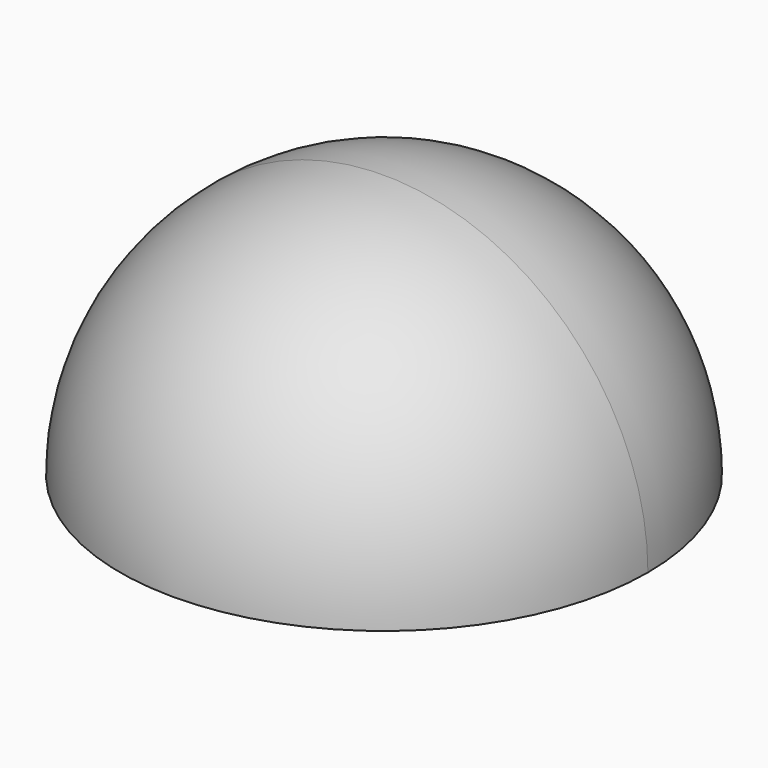
from build123d import *

# Parameters (mm, degrees)
F1_ANGLE = 180


with BuildPart() as f1:
    # F0 (on Top) → F1 (revolve)
    with BuildSketch(Plane.XY):
        with BuildLine():
            ThreePointArc((0, -31.75), (22.4506403027, -22.4506403027), (31.75, 0))
            ThreePointArc((31.75, 0), (22.4506403027, 22.4506403027), (0, 31.75))
            Line((0, 31.75), (0, 25.4))
            ThreePointArc((0, 25.4), (17.9605122421, 17.9605122421), (25.4, 0))
            ThreePointArc((25.4, 0), (17.9605122421, -17.9605122421), (0, -25.4))
            Line((0, -25.4), (0, -31.75))
        make_face()
    revolve(axis=Axis((0, 0, 0), (0, -1, 0)), revolution_arc=F1_ANGLE)


solid = f1.part
